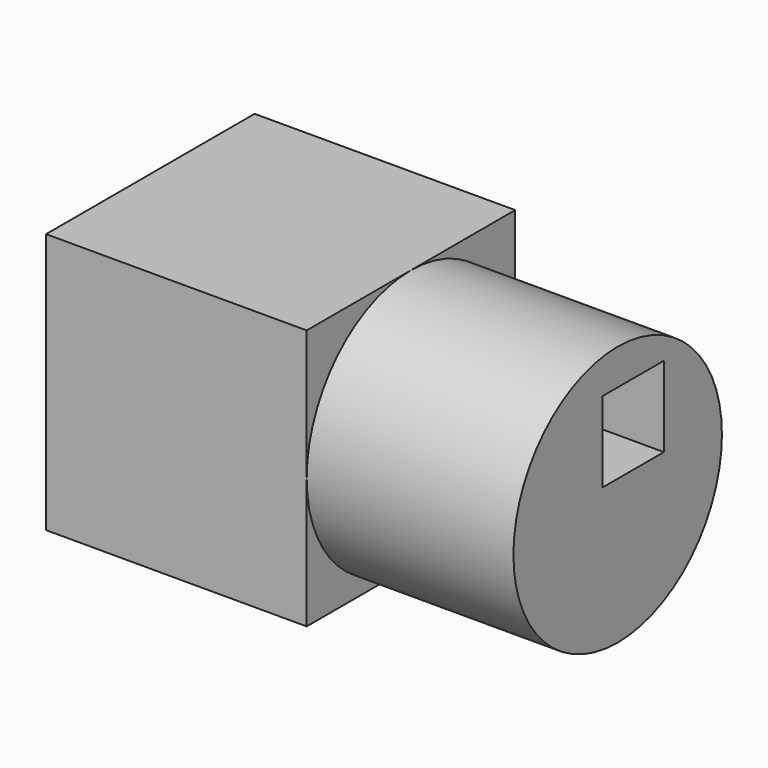
from build123d import *

# Parameters (mm, degrees)
F1_W     = 38.1
F1_H     = 38.1
F2_DEPTH = 19.05
F3_R     = 19.05
F4_DEPTH = 30.226
F5_W     = 11.2522
F5_H     = 11.7586595006
F6_DEPTH = 68.327


# Not quite as in the source:
# - a variable given as a bare number and used for a length is read in inches; the dataset says mm whatever the document's units were


with BuildPart() as f2:
    # F1 (on Front) → F2 (new body, symmetric)
    with BuildSketch(Plane.XZ):
        Rectangle(F1_W, F1_H)
    extrude(amount=F2_DEPTH, both=True)

    # F3 (on face) → F4 (join)
    with BuildSketch(Plane.YZ.offset(19.05)):
        Circle(F3_R)
    extrude(amount=F4_DEPTH)

    # F5 (on face) → F6 (cut, through all)
    with BuildSketch(Plane.YZ.offset(49.276)):
        with Locations((2.8142485544, 7.924313657)):
            Rectangle(F5_W, F5_H)
    extrude(amount=-F6_DEPTH, mode=Mode.SUBTRACT)


solid = f2.part
